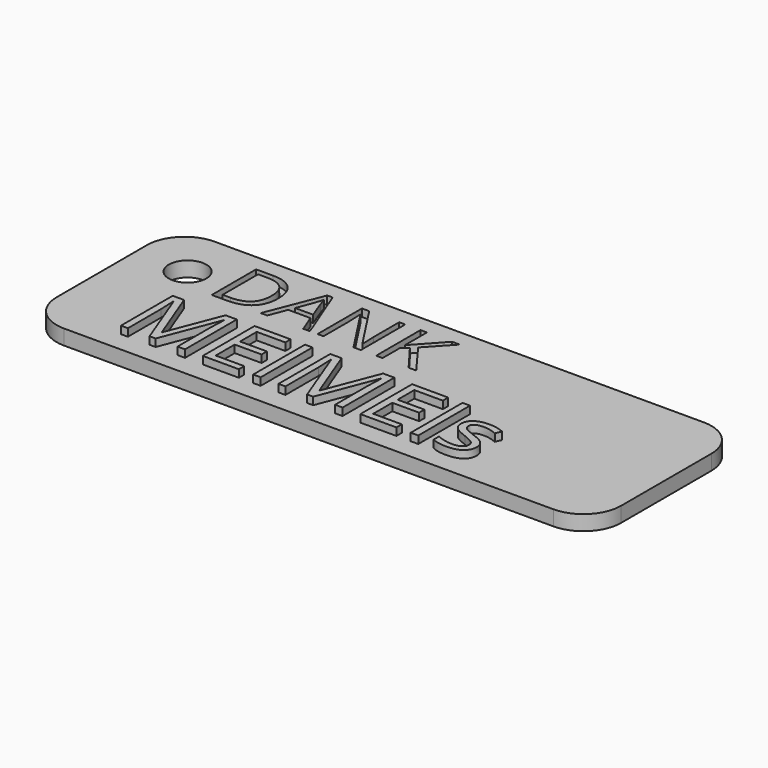
from build123d import *

# Parameters (mm, degrees)
F1_DEPTH     = 2
F3_D         = 5
F4_TEXT_SIZE = 10.323743724
F5_DEPTH     = 1
F6_TEXT_SIZE = 12.0458392646
F7_DEPTH     = 1


# Not quite as in the source:
# - Text() gives the source's letters only with a copy of the font that has no kerning and outlines rounded to 1/6400 em; it was checked with that copy


with BuildPart() as f1:
    # F0 (on Top) → F1 (new body)
    with BuildSketch(Plane.XY):
        with BuildLine():
            Line((32.5, 12.5), (-32.5, 12.5))
            ThreePointArc((-32.5, 12.5), (-36.0355339059, 11.0355339059), (-37.5, 7.5))
            Line((-37.5, 7.5), (-37.5, -7.5))
            ThreePointArc((-37.5, -7.5), (-36.0355339059, -11.0355339059), (-32.5, -12.5))
            Line((-32.5, -12.5), (32.5, -12.5))
            ThreePointArc((32.5, -12.5), (36.0355339059, -11.0355339059), (37.5, -7.5))
            Line((37.5, -7.5), (37.5, 7.5))
            ThreePointArc((37.5, 7.5), (36.0355339059, 11.0355339059), (32.5, 12.5))
        make_face()
    extrude(amount=F1_DEPTH)

    # F3 (through all)
    with Locations(Plane.XY.offset(2)):
        with Locations((-30.5, 5.5)):
            Hole(F3_D / 2)

    # F4 (on face) → F5 (cut)
    with BuildSketch(Plane.XY.offset(2)):
        with Locations((-26.2673702091, 2.955976408)):
            Text('DANK', F4_TEXT_SIZE, font='Open Sans', text_align=(TextAlign.LEFT, TextAlign.BOTTOM))
    extrude(amount=-F5_DEPTH, mode=Mode.SUBTRACT)

    # F6 (on face) → F7 (join)
    with BuildSketch(Plane.XY.offset(2)):
        with Locations((-28.2836662909, -9.812616033)):
            Text('MEIMEIs', F6_TEXT_SIZE, font='Open Sans', text_align=(TextAlign.LEFT, TextAlign.BOTTOM))
    extrude(amount=F7_DEPTH)


solid = f1.part
